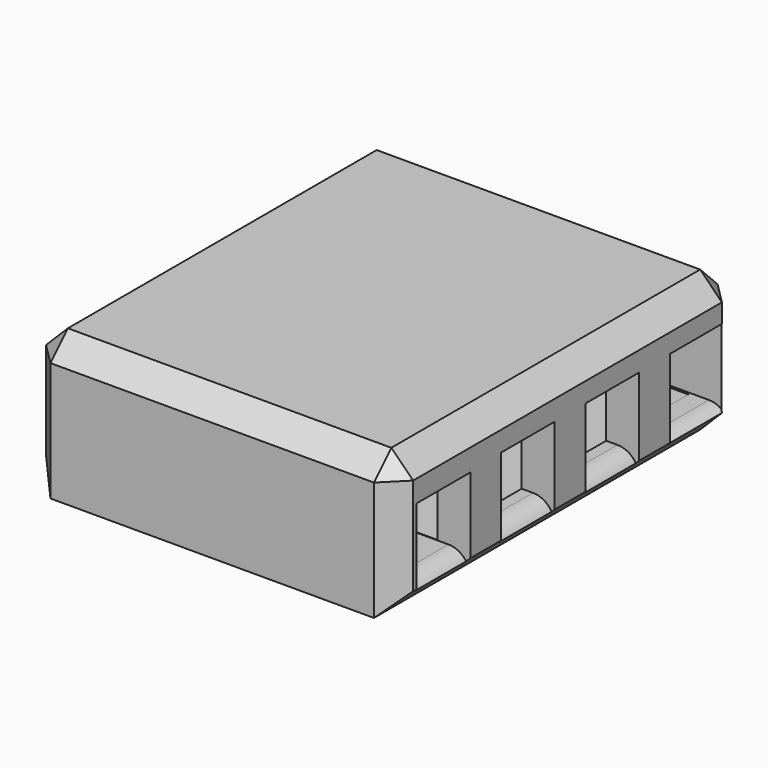
from build123d import *

# Parameters (mm, degrees)
F1_W          = 85.6011658907
F1_H          = 100.1833304763
F1_W_2        = 68.7451
F1_H_2        = 88.9635
F2_DEPTH      = 23.9903
F3_W          = 88.7990454212
F3_H          = 23.9903
F4_DEPTH      = 25.4
F5_W          = 85.6011658907
F5_H          = 100.1833304763
F6_DEPTH      = 6.35
F7_W          = 85.6011658907
F7_H          = 100.1833304763
F8_DEPTH      = 2.54
F10_W         = 34.5417858863
F10_H         = 14.8036217375
F11_DEPTH     = 25.4
F9_W          = 15.6851452775
F9_H          = 16.9501625933
F9_H_2        = 16.5283605456
F9_H_3        = 16.275445465
F9_H_4        = 16.4441019297
F12_DEPTH     = 25.4
F13_T1_DEPTH  = 6.4524666085
F13_T3_DEPTH  = 6.4524666085
F13_T5_DEPTH  = 6.4524666085
F13_T7_DEPTH  = 6.4524666085
F13_T9_DEPTH  = 6.4524666085
F13_T11_DEPTH = 6.4524666085
F13_T13_DEPTH = 111.7294650484
F13_T15_DEPTH = 126.311629634
F13_T17_DEPTH = 59.0085991577
F14_T1_DEPTH  = 34.5417858863
F14_T3_DEPTH  = 15.6851452775
F14_T5_DEPTH  = 15.6851452775
F14_T7_DEPTH  = 15.6851452775
F14_T9_DEPTH  = 88.7990454212
F14_T14_DEPTH = 23.7610080402
F14_T19_DEPTH = 41.0851452775
F14_T24_DEPTH = 41.0851452775


# Not quite as in the source:
# - a fillet or chamfer that OpenCascade refuses, or shapes differently, is made with other operations: its cross-section is extruded or revolved along the edge and cut away or added


with BuildPart() as f2:
    # F1 (on face) → F2 (new body)
    with BuildSketch(Plane.XY):
        with Locations((-5.5697076023, 30.5755026639)):
            Rectangle(F1_W, F1_H)
        with Locations((-4.8453267664, 31.0760242272)):
            Rectangle(F1_W_2, F1_H_2, mode=Mode.SUBTRACT)
    extrude(amount=-F2_DEPTH)

    # F3 (on face) → F4 (cut)
    with BuildSketch(Plane(origin=(-48.3702905476, 0, 0), x_dir=(0, -1, 0), z_dir=(-1, 0, 0))):
        with Locations((-31.1722527258, -11.99515)):
            Rectangle(F3_W, F3_H)
    extrude(amount=-F4_DEPTH, mode=Mode.SUBTRACT)

    # F5 (on face) → F6 (join)
    with BuildSketch(Plane(origin=(0, 0, -23.9903), x_dir=(1, 0, 0), z_dir=(0, 0, -1))):
        with Locations((-5.5697076023, -30.5755026639)):
            Rectangle(F5_W, F5_H)
    extrude(amount=F6_DEPTH)

    # F7 (on face) → F8 (join)
    with BuildSketch(Plane.XY):
        with Locations((-5.5697076023, 30.5755026639)):
            Rectangle(F7_W, F7_H)
    extrude(amount=F8_DEPTH)

    # F10 (on face) → F11 (cut)
    with BuildSketch(Plane(origin=(0, 80.667167902, 0), x_dir=(-1, 0, 0), z_dir=(0, 1, 0))):
        with Locations((17.8098176001, -14.4762154669)):
            Rectangle(F10_W, F10_H)
    extrude(amount=-F11_DEPTH, mode=Mode.SUBTRACT)

    # F9 (on face) → F12 (cut)
    with BuildSketch(Plane.YZ.offset(37.2308753431)):
        with Locations((68.261611322, -15.4458589386)):
            Rectangle(F9_W, F9_H)
        with Locations((43.6356660444, -15.403628815)):
            Rectangle(F9_W, F9_H_2)
        with Locations((19.0097207669, -15.3615369927)):
            Rectangle(F9_W, F9_H_3)
        with Locations((-5.614269292, -15.8675089478)):
            Rectangle(F9_W, F9_H_4)
    extrude(amount=-F12_DEPTH, mode=Mode.SUBTRACT)

    # F13: chamfer of 5.08 on 11 edges, made by hand

    # F13_s2 → F13_t1 (cut)
    with BuildSketch(Plane(origin=(36.7593477484, 36.7593477484, 36.7593477484), x_dir=(-0.7071067812, 0.7071067812, 0), z_dir=(0.5773502692, 0.5773502692, 0.5773502692))):
        Polygon((27.1219945696, -48.1316746038), (30.714097018, -41.9099706572), (34.3061994664, -48.1316746038), align=None)
    extrude(amount=F13_T1_DEPTH, mode=Mode.SUBTRACT)

    # F13_s4 → F13_t3 (cut)
    with BuildSketch(Plane(origin=(-40.4724861499, 40.4724861499, 40.4724861499), x_dir=(-0.7071067812, -0.7071067812, 0), z_dir=(-0.5773502692, 0.5773502692, 0.5773502692))):
        Polygon((-19.24523854, -52.6793218179), (-22.8373409884, -46.4576178712), (-26.4294434369, -52.6793218179), align=None)
    extrude(amount=F13_T3_DEPTH, mode=Mode.SUBTRACT)

    # F13_s6 → F13_t5 (cut)
    with BuildSketch(Plane(origin=(16.3756793058, -16.3756793058, 16.3756793058), x_dir=(0.7071067812, 0.7071067812, 0), z_dir=(0.5773502692, -0.5773502692, 0.5773502692))):
        Polygon((16.118295974, -23.1668812187), (8.9340910772, -23.1668812187), (12.5261935256, -16.945177272), align=None)
    extrude(amount=F13_T5_DEPTH, mode=Mode.SUBTRACT)

    # F13_s8 → F13_t7 (cut)
    with BuildSketch(Plane(origin=(-20.0888177073, -20.0888177073, 20.0888177073), x_dir=(0.7071067812, -0.7071067812, 0), z_dir=(-0.5773502692, -0.5773502692, 0.5773502692))):
        Polygon((-23.9950520036, -27.7145284327), (-16.8108471067, -27.7145284327), (-20.4029495552, -21.492824486), align=None)
    extrude(amount=F13_T7_DEPTH, mode=Mode.SUBTRACT)

    # F13_s10 → F13_t9 (cut)
    with BuildSketch(Plane(origin=(-49.7392528165, 49.7392528165, -49.7392528165), x_dir=(-0.7071067812, -0.7071067812, 0), z_dir=(-0.5773502692, 0.5773502692, -0.5773502692))):
        Polygon((-19.24523854, 29.9804719191), (-22.8373409884, 23.7587679724), (-26.4294434369, 29.9804719191), align=None)
    extrude(amount=F13_T9_DEPTH, mode=Mode.SUBTRACT)

    # F13_s12 → F13_t11 (cut)
    with BuildSketch(Plane(origin=(46.026114415, 46.026114415, -46.026114415), x_dir=(-0.7071067812, 0.7071067812, 0), z_dir=(0.5773502692, 0.5773502692, -0.5773502692))):
        Polygon((27.1219945696, 25.4328247051), (34.3061994664, 25.4328247051), (30.714097018, 19.2111207584), align=None)
    extrude(amount=F13_T11_DEPTH, mode=Mode.SUBTRACT)

    # F13_s14 → F13_t13 (cut)
    with BuildSketch(Plane.YZ.offset(-61.4344401265)):
        Polygon((75.587167902, 2.54), (80.667167902, -2.54), (80.667167902, 2.54), align=None)
        Polygon((-19.5161625743, -2.54), (-14.4361625743, 2.54), (-19.5161625743, 2.54), align=None)
        Polygon((75.587167902, -30.3403), (80.667167902, -25.2603), (80.667167902, -30.3403), align=None)
    extrude(amount=F13_T13_DEPTH, mode=Mode.SUBTRACT)

    # F13_s16 → F13_t15 (cut)
    with BuildSketch(Plane.XZ.offset(-93.7313174809)):
        Polygon((32.1508753431, 2.54), (37.2308753431, -2.54), (37.2308753431, 2.54), align=None)
        Polygon((-48.3702905476, -2.54), (-43.2902905476, 2.54), (-48.3702905476, 2.54), align=None)
        Polygon((-48.3702905476, -25.2603), (-43.2902905476, -30.3403), (-48.3702905476, -30.3403), align=None)
        Polygon((32.1508753431, -30.3403), (37.2308753431, -25.2603), (37.2308753431, -30.3403), align=None)
    extrude(amount=F13_T15_DEPTH, mode=Mode.SUBTRACT)

    # F13_s18 → F13_t17 (cut)
    with BuildSketch(Plane.XY.offset(-43.4044495789)):
        Polygon((-48.3702905476, -14.4361625743), (-43.2902905476, -19.5161625743), (-48.3702905476, -19.5161625743), align=None)
        Polygon((-48.3702905476, 75.587167902), (-43.2902905476, 80.667167902), (-48.3702905476, 80.667167902), align=None)
        Polygon((32.1508753431, 80.667167902), (37.2308753431, 75.587167902), (37.2308753431, 80.667167902), align=None)
        Polygon((32.1508753431, -19.5161625743), (37.2308753431, -14.4361625743), (37.2308753431, -19.5161625743), align=None)
    extrude(amount=F13_T17_DEPTH, mode=Mode.SUBTRACT)

    # F14: fillet of radius 5.08 on 6 edges, made by hand

    # F14_s2 → F14_t1 (cut)
    with BuildSketch(Plane.YZ.offset(-35.0807105432)):
        with BuildLine():
            ThreePointArc((80.667167902, -26.9580263356), (79.1792703504, -23.3659238872), (75.587167902, -21.8780263356))
            Line((75.587167902, -21.8780263356), (80.667167902, -21.8780263356))
            Line((80.667167902, -21.8780263356), (80.667167902, -26.9580263356))
        make_face()
    extrude(amount=F14_T1_DEPTH, mode=Mode.SUBTRACT)

    # F14_s4 → F14_t3 (cut)
    with BuildSketch(Plane.XZ.offset(-51.4782386832)):
        with BuildLine():
            ThreePointArc((37.2308753431, -28.7478090878), (35.7429777915, -25.1557066394), (32.1508753431, -23.6678090878))
            Line((32.1508753431, -23.6678090878), (37.2308753431, -23.6678090878))
            Line((37.2308753431, -23.6678090878), (37.2308753431, -28.7478090878))
        make_face()
    extrude(amount=F14_T3_DEPTH, mode=Mode.SUBTRACT)

    # F14_s6 → F14_t5 (cut)
    with BuildSketch(Plane.XZ.offset(-26.8522934057)):
        with BuildLine():
            ThreePointArc((37.2308753431, -28.5792597252), (35.7429777915, -24.9871572768), (32.1508753431, -23.4992597252))
            Line((32.1508753431, -23.4992597252), (37.2308753431, -23.4992597252))
            Line((37.2308753431, -23.4992597252), (37.2308753431, -28.5792597252))
        make_face()
    extrude(amount=F14_T5_DEPTH, mode=Mode.SUBTRACT)

    # F14_s8 → F14_t7 (cut)
    with BuildSketch(Plane.XZ.offset(-2.2283033468)):
        with BuildLine():
            ThreePointArc((32.1508753431, -24.0895599127), (35.7429777915, -25.5774574643), (37.2308753431, -29.1695599127))
            Line((37.2308753431, -29.1695599127), (37.2308753431, -24.0895599127))
            Line((37.2308753431, -24.0895599127), (32.1508753431, -24.0895599127))
        make_face()
    extrude(amount=F14_T7_DEPTH, mode=Mode.SUBTRACT)

    # F14_s10 → F14_t9 (cut)
    with BuildSketch(Plane.XZ.offset(-75.5717754364)):
        with BuildLine():
            ThreePointArc((-48.3702905476, -29.0703), (-46.882392996, -25.4781975516), (-43.2902905476, -23.9903))
            Line((-43.2902905476, -23.9903), (-48.3702905476, -23.9903))
            Line((-48.3702905476, -23.9903), (-48.3702905476, -29.0703))
        make_face()
    extrude(amount=F14_T9_DEPTH, mode=Mode.SUBTRACT)


with BuildPart() as f14_tool12:
    # F14_s13 → F14_t14 (new body)
    with BuildSketch(Plane.XZ.offset(-60.4190386832)):
        with BuildLine():
            ThreePointArc((37.2308753431, -25.2603), (35.6381678507, -24.2676088294), (33.7937238145, -23.9209402353))
            Line((33.7937238145, -23.9209402353), (37.2308753431, -23.9209402353))
            Line((37.2308753431, -23.9209402353), (37.2308753431, -25.2603))
        make_face()
    extrude(amount=-F14_T14_DEPTH)

    split(bisect_by=Plane.XZ.offset(-76.1041839607), keep=Keep.TOP)


with BuildPart() as f2_1:
    add(f2.part)

    # F14_t11: cut F14_tool12
    add(f14_tool12.part, mode=Mode.SUBTRACT)


with BuildPart() as f14_tool17:
    # F14_s18 → F14_t19 (new body)
    with BuildSketch(Plane.XZ.offset(1.5328518718)):
        with BuildLine():
            ThreePointArc((37.2308753431, -28.5792597252), (35.7429777915, -24.9871572768), (32.1508753431, -23.4992597252))
            Line((32.1508753431, -23.4992597252), (37.2308753431, -23.4992597252))
            Line((37.2308753431, -23.4992597252), (37.2308753431, -28.5792597252))
        make_face()
    extrude(amount=-F14_T19_DEPTH)

    split(bisect_by=Plane.XZ.offset(-2.2283033468), keep=Keep.TOP)


with BuildPart() as f2_2:
    add(f2_1.part)

    # F14_t16: cut F14_tool17
    add(f14_tool17.part, mode=Mode.SUBTRACT)


with BuildPart() as f14_tool22:
    # F14_s23 → F14_t24 (new body)
    with BuildSketch(Plane.XZ.offset(1.5328518718)):
        with BuildLine():
            ThreePointArc((37.2308753431, -28.5792597252), (35.7429777915, -24.9871572768), (32.1508753431, -23.4992597252))
            Line((32.1508753431, -23.4992597252), (37.2308753431, -23.4992597252))
            Line((37.2308753431, -23.4992597252), (37.2308753431, -28.5792597252))
        make_face()
    extrude(amount=-F14_T24_DEPTH)

    split(bisect_by=Plane.XZ.offset(-35.7930934057), keep=Keep.BOTTOM)


with BuildPart() as f2_3:
    add(f2_2.part)

    # F14_t21: cut F14_tool22
    add(f14_tool22.part, mode=Mode.SUBTRACT)


solid = f2_3.part
